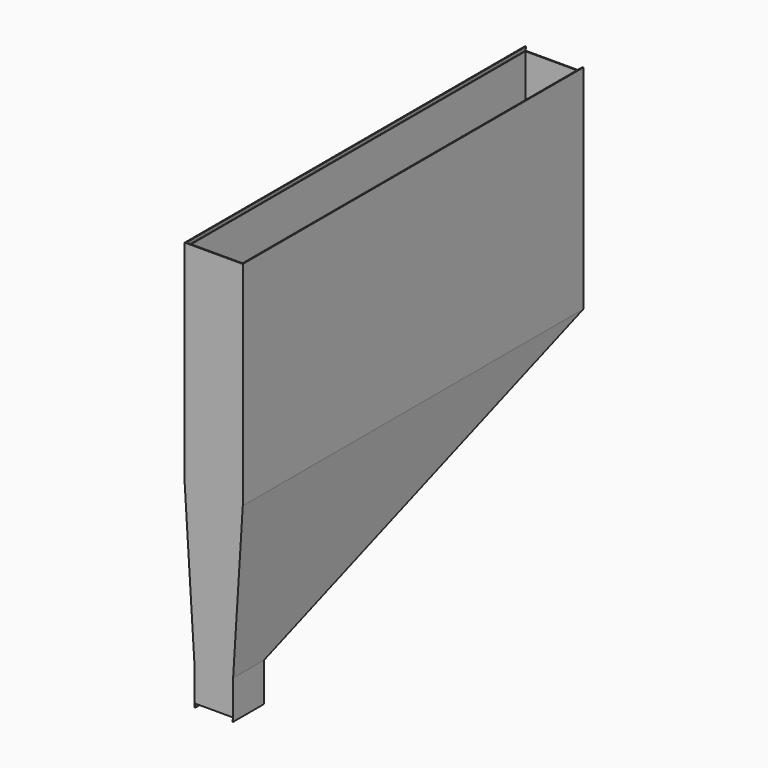
from build123d import *

# Parameters (mm, degrees)
F0_W        = 100
F0_H        = 100
F0_W_2      = 150
F0_H_2      = 550
F1_DEPTH    = 550
F3_DEPTH    = 150
F4_T        = 2.5
F4_T3_DEPTH = 105
F4_T5_DEPTH = 105
F6_DEPTH    = 98.5
F7_W        = 145
F7_H        = 5
F8_DEPTH    = 2.5
F9_DEPTH    = 1099


# Not quite as in the source:
# - a shell that OpenCascade refuses in one call is made with other operations: the cavity is built on its own and cut out


with BuildPart() as f1:
    # F0 (on Front) → F1 (new body, symmetric)
    with BuildSketch(Plane.XZ):
        with Locations((0, -450)):
            Rectangle(F0_W, F0_H)
        with Locations((0, 275)):
            Rectangle(F0_W_2, F0_H_2)
        Polygon((75, 0), (-75, 0), (-50, -400), (50, -400), align=None)
    extrude(amount=F1_DEPTH, both=True)

    # F2 (on face) → F3 (cut)
    with BuildSketch(Plane.YZ.offset(75)):
        Polygon((550, -500), (550, 0), (-450, -400), (-450, -500), align=None)
    extrude(amount=-F3_DEPTH, mode=Mode.SUBTRACT)

    # F4: shell of thickness 2.5, made by hand


with BuildPart() as f4_core1:
    # F4_t2: copy of F1
    add(f1.part)

    # the walls: a layer under each face that stays
    f4_faces = [f4_core1.faces().sort_by_distance(p)[0] for p in [
        (-50, -500, -450),
        (-62.5, 0, -200),
        (0, -550, 25),
        (0, -450, -450),
        (-75, 0, 275),
        (0, 50, -200),
        (50, -500, -450),
        (62.5, 0, -200),
        (75, 0, 275),
        (0, 550, 275),
    ]]
    thicken(f4_faces, amount=-F4_T, mode=Mode.SUBTRACT)

    # F4_s4 → F4_t3 (cut)
    with BuildSketch(Plane.XZ.offset(447.5)):
        Polygon((-50.0499513145, -400.0015594572), (-47.5, -400), (-47.5, -399.9219511453), (-47.5048685538, -399.8440542846), align=None)
        Polygon((50.0499513145, -400.0015594572), (47.5, -400), (47.5, -399.9219511453), (47.5048685538, -399.8440542846), align=None)
    extrude(amount=F4_T3_DEPTH, mode=Mode.SUBTRACT)

    # F4_s6 → F4_t5 (cut)
    with BuildSketch(Plane.YZ.offset(-52.5)):
        Polygon((-449.9657152331, -400.0232119173), (-452.5, -400), (-452.5, -398.3074175964), (-450.9284766909, -397.6788082728), align=None)
    extrude(amount=F4_T5_DEPTH, mode=Mode.SUBTRACT)


with BuildPart() as f1_1:
    add(f1.part)

    # what is left inside the walls is the cavity
    f4_cavity = [f4_core1.part.solids().sort_by_distance(p)[0] for p in [
        (-72.475, 182.5, 275.039024),
    ]]
    add(f4_cavity, mode=Mode.SUBTRACT)

    # F5 (on face) → F6 (cut)
    with BuildSketch(Plane.XZ.offset(550)):
        Polygon((-48.5, -495), (-48.5, -500), (48.5, -500), (48.5, -495), (49.5, -495), (49.5, -490), (-49.5, -490), (-49.5, -495), align=None)
    extrude(amount=-F6_DEPTH, mode=Mode.SUBTRACT)

    # F7 (on face) → F8 (cut)
    with BuildSketch(Plane(origin=(0, 550, 0), x_dir=(-1, 0, 0), z_dir=(0, 1, 0))):
        with Locations((0, 547.5)):
            Rectangle(F7_W, F7_H)
    extrude(amount=-F8_DEPTH, mode=Mode.SUBTRACT)

    # F7 (on face) → F9 (cut)
    with BuildSketch(Plane(origin=(0, 550, 0), x_dir=(-1, 0, 0), z_dir=(0, 1, 0))):
        Polygon((-74, 545), (-74, 540), (74, 540), (74, 545), (72.5, 545), (-72.5, 545), align=None)
    extrude(amount=-F9_DEPTH, mode=Mode.SUBTRACT)


solid = f1_1.part
